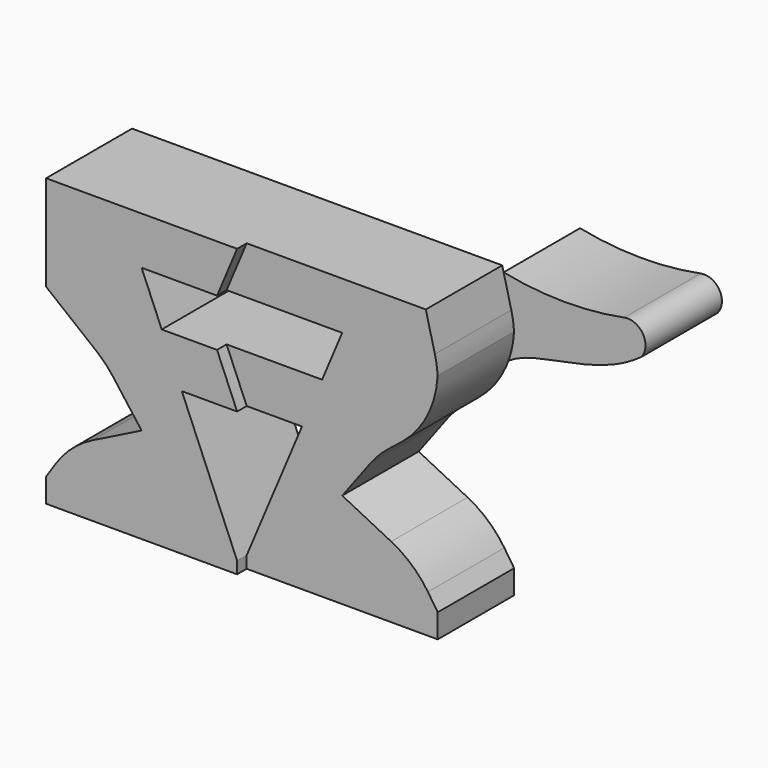
from build123d import *

# Parameters (mm, degrees)
F1_DEPTH    = 25.4
F2_T1_DEPTH = 25.4
F2_T3_DEPTH = 41.0344144534
F2_T5_DEPTH = 86.4393556308
F2_T7_DEPTH = 59.1266835085
F4_DEPTH    = 25.4
F6_DEPTH    = 50.8010001
F8_DEPTH    = 3.175
F9_R        = 25.4


# Not quite as in the source:
# - a fillet or chamfer that OpenCascade refuses, or shapes differently, is made with other operations: its cross-section is extruded or revolved along the edge and cut away or added


with BuildPart() as f1:
    # F0 (on Front) → F1 (new body)
    with BuildSketch(Plane.XZ):
        Polygon((-50.8, -38.1), (50.8, -38.1), (50.8, -31.75), (44.45, -22.225), (25.4, -12.7), (34.925, 0), (50.8, 12.7), (50.8, 25.4), (47.625, 38.1), (-50.8, 38.1), (-50.8, 12.7), (-34.925, 0), (-25.4, -12.7), (-44.45, -22.225), (-50.8, -31.75), align=None)
    extrude(amount=F1_DEPTH)

    # F2: fillet of radius 25.4 on 4 edges, made by hand

    # F2_s2 → F2_t1 (join)
    with BuildSketch(Plane.XZ):
        with BuildLine():
            ThreePointArc((32.9902416385, -2.5796778154), (35.0713900731, -0.1418868454), (37.4429874306, 2.0143899445))
            Line((37.4429874306, 2.0143899445), (34.925, 0))
            Line((34.925, 0), (32.9902416385, -2.5796778154))
        make_face()
    extrude(amount=F2_T1_DEPTH)

    # F2_s4 → F2_t3 (cut)
    with BuildSketch(Plane.XZ.offset(-7.8172072267)):
        with BuildLine():
            ThreePointArc((50.8, 22.2731171093), (50.6096919397, 25.3765720072), (50.0416195037, 28.4335219852))
            Line((50.0416195037, 28.4335219852), (50.8, 25.4))
            Line((50.8, 25.4), (50.8, 22.2731171093))
        make_face()
    extrude(amount=F2_T3_DEPTH, mode=Mode.SUBTRACT)

    # F2_s6 → F2_t5 (cut)
    with BuildSketch(Plane.XZ.offset(-30.5196778154)):
        with BuildLine():
            ThreePointArc((41.2672542079, 5.0738033663), (48.2931022022, 13.9048773717), (50.8, 24.9078711262))
            Line((50.8, 24.9078711262), (50.8, 12.7))
            Line((50.8, 12.7), (41.2672542079, 5.0738033663))
        make_face()
    extrude(amount=F2_T5_DEPTH, mode=Mode.SUBTRACT)

    # F2_s8 → F2_t7 (cut)
    with BuildSketch(Plane.XZ.offset(-16.8633417542)):
        with BuildLine():
            ThreePointArc((48.191639592, -27.8374593881), (43.867347222, -22.8850187065), (38.4167874416, -19.2083937208))
            Line((38.4167874416, -19.2083937208), (44.45, -22.225))
            Line((44.45, -22.225), (48.191639592, -27.8374593881))
        make_face()
    extrude(amount=F2_T7_DEPTH, mode=Mode.SUBTRACT)

    # F5 (on face) → F6 (cut, through all)
    with BuildSketch(Plane.XZ.offset(25.4)):
        Polygon((25.4, 25.4), (-25.4, 25.4), (-20.0526315789, 12.7), (20.0526315789, 12.7), align=None)
        Polygon((14.7052631579, 0), (-14.7052631579, 0), (0, -34.925), align=None)
    extrude(amount=-F6_DEPTH, mode=Mode.SUBTRACT)

    # F7 (on face) → F8 (join)
    with BuildSketch(Plane.XZ.offset(25.4)):
        Polygon((-14.7052631579, 0), (0, 0), (-5.3473684211, 12.7), (-20.0526315789, 12.7), (-25.4, 25.4), (-5.3473684211, 25.4), (0, 38.1), (-50.8, 38.1), (-50.8, 12.7), (-34.925, 0), (-25.4, -12.7), (-44.45, -22.225), (-50.8, -31.75), (-50.8, -38.1), (0, -38.1), (0, -34.925), align=None)
    extrude(amount=F8_DEPTH)

    # F9
    f9_edges = [f1.edges().sort_by_distance(p)[0] for p in [
        (-34.925, -14.2875, 0),
        (-44.45, -14.2875, -22.225),
    ]]
    fillet(f9_edges, radius=F9_R)


with BuildPart() as f4:
    # F3 (on face) → F4 (new body)
    with BuildSketch(Plane(origin=(0, 0, 0), x_dir=(-1, 0, 0), z_dir=(0, 1, 0))):
        with BuildLine():
            ThreePointArc((-48.0006987759, 36.5972048963), (-64.0191987714, 34.9261782663), (-80.0547112422, 36.4251819025))
            ThreePointArc((-80.0547112422, 36.4251819025), (-85.0772133008, 34.1480285032), (-84.5827576486, 28.6556275583))
            add(Edge.make_bspline(
                [(-82.4520441677, 27.2264323347), (-83.1820950721, 27.6822920244), (-83.8902700056, 28.1587482087), (-84.5827576486, 28.6556275583)],
                knots=[0.9280008954, 0.9280008954, 0.9280008954, 0.9280008954, 1, 1, 1, 1], degree=3))
            add(Edge.make_bspline(
                [(-49.3181387168, 16.3590325895), (-51.4536007413, 17.6963242827), (-56.3528215031, 19.6709837112), (-72.2028273002, 22.0187338367), (-79.6974095968, 25.5063784956), (-82.4520441677, 27.2264323347)],
                knots=[0, 0, 0, 0, 0.2639502882, 0.6563332329, 0.9280008954, 0.9280008954, 0.9280008954, 0.9280008954], degree=3))
            ThreePointArc((-49.3181387168, 16.3590325895), (-50.3058327868, 19.9219416041), (-50.7658139593, 23.5904941174))
            ThreePointArc((-50.7658139593, 23.5904941174), (-50.5207002315, 26.0295009926), (-50.0416195037, 28.4335219852))
            Line((-50.0416195037, 28.4335219852), (-48.0006987759, 36.5972048963))
        make_face()
    extrude(amount=F4_DEPTH)


solid = Compound([f1.part, f4.part])
